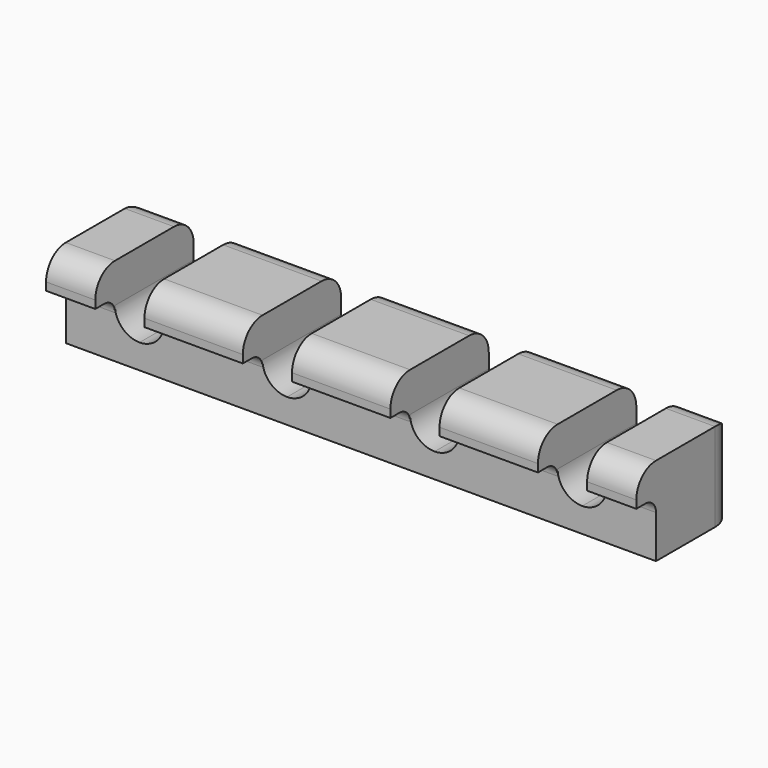
from build123d import *

# Parameters (mm, degrees)
F0_W      = 76.2
F0_H      = 12.7
F1_DEPTH  = 3.175
F2_W      = 6.35
F2_H      = 12.7
F2_W_2    = 12.7
F3_DEPTH  = 8.255
F4_W      = 6.35
F4_H      = 4.191
F4_W_2    = 12.7
F5_DEPTH  = 3.175
F7_DEPTH  = 6.35
F9_DEPTH  = 12.7
F11_DEPTH = 12.7
F13_DEPTH = 12.7
F15_DEPTH = 6.35
F17_DEPTH = 12.7
F18_R     = 3.175


with BuildPart() as f1:
    # F0 (on Top) → F1 (new body)
    with BuildSketch(Plane.XY):
        with Locations((-12.1522513986, 0.3075693393)):
            Rectangle(F0_W, F0_H)
    extrude(amount=F1_DEPTH)

    # F2 (on face) → F3 (join)
    with BuildSketch(Plane.XY.offset(3.175)):
        with Locations((-47.0772513986, 0.3075693393)):
            Rectangle(F2_W, F2_H)
        with Locations((-31.2022513986, 0.3075693393)):
            Rectangle(F2_W_2, F2_H)
        with Locations((-12.1522513986, 0.3075693393)):
            Rectangle(F2_W_2, F2_H)
        with Locations((6.8977486014, 0.3075693393)):
            Rectangle(F2_W_2, F2_H)
        with Locations((22.7727486014, 0.3075693393)):
            Rectangle(F2_W, F2_H)
    extrude(amount=F3_DEPTH)

    # F4 (on face) → F5 (join)
    with BuildSketch(Plane.XZ.offset(6.0424306607)):
        with Locations((-47.0772513986, 9.3345)):
            Rectangle(F4_W, F4_H)
        with Locations((-31.2022513986, 9.3345)):
            Rectangle(F4_W_2, F4_H)
        with Locations((-12.1522513986, 9.3345)):
            Rectangle(F4_W_2, F4_H)
        with Locations((6.8977486014, 9.3345)):
            Rectangle(F4_W_2, F4_H)
        with Locations((22.7727486014, 9.3345)):
            Rectangle(F4_W, F4_H)
    extrude(amount=F5_DEPTH)

    # F6 (on face) → F7 (join)
    with BuildSketch(Plane.YZ.offset(25.9477486014)):
        with BuildLine():
            Line((-6.0424306607, 7.239), (-7.7569306607, 7.239))
            ThreePointArc((-7.7569306607, 7.239), (-6.5445960844, 6.7368345763), (-6.0424306607, 5.5245))
            Line((-6.0424306607, 5.5245), (-6.0424306607, 7.239))
        make_face()
    extrude(amount=-F7_DEPTH)

    # F8 (on face) → F9 (join)
    with BuildSketch(Plane.YZ.offset(13.2477486014)):
        with BuildLine():
            Line((-6.0424306607, 7.239), (-7.7569306607, 7.239))
            ThreePointArc((-7.7569306607, 7.239), (-6.5445960844, 6.7368345763), (-6.0424306607, 5.5245))
            Line((-6.0424306607, 5.5245), (-6.0424306607, 7.239))
        make_face()
    extrude(amount=-F9_DEPTH)

    # F10 (on face) → F11 (join)
    with BuildSketch(Plane.YZ.offset(-5.8022513986)):
        with BuildLine():
            Line((-6.0424306607, 7.239), (-7.7569306607, 7.239))
            ThreePointArc((-7.7569306607, 7.239), (-6.5445960844, 6.7368345763), (-6.0424306607, 5.5245))
            Line((-6.0424306607, 5.5245), (-6.0424306607, 7.239))
        make_face()
    extrude(amount=-F11_DEPTH)

    # F12 (on face) → F13 (join)
    with BuildSketch(Plane.YZ.offset(-24.8522513986)):
        with BuildLine():
            Line((-6.0424306607, 7.239), (-7.7569306607, 7.239))
            ThreePointArc((-7.7569306607, 7.239), (-6.5445960844, 6.7368345763), (-6.0424306607, 5.5245))
            Line((-6.0424306607, 5.5245), (-6.0424306607, 7.239))
        make_face()
    extrude(amount=-F13_DEPTH)

    # F14 (on face) → F15 (join)
    with BuildSketch(Plane.YZ.offset(-43.9022513986)):
        with BuildLine():
            Line((-6.0424306607, 7.239), (-7.7569306607, 7.239))
            ThreePointArc((-7.7569306607, 7.239), (-6.5445960844, 6.7368345763), (-6.0424306607, 5.5245))
            Line((-6.0424306607, 5.5245), (-6.0424306607, 7.239))
        make_face()
    extrude(amount=-F15_DEPTH)

    # F16 (on face) → F17 (join)
    with BuildSketch(Plane.XZ.offset(6.0424306607)):
        with BuildLine():
            ThreePointArc((-40.7272513986, 3.175), (-42.9723154288, 4.1049359697), (-43.9022513986, 6.35))
            Line((-43.9022513986, 6.35), (-43.9022513986, 5.5245))
            Line((-43.9022513986, 5.5245), (-43.9022513986, 3.175))
            Line((-43.9022513986, 3.175), (-40.7272513986, 3.175))
        make_face()
        with BuildLine():
            ThreePointArc((-37.5522513986, 6.35), (-38.4821873683, 4.1049359697), (-40.7272513986, 3.175))
            Line((-40.7272513986, 3.175), (-37.5522513986, 3.175))
            Line((-37.5522513986, 3.175), (-37.5522513986, 5.5245))
            Line((-37.5522513986, 5.5245), (-37.5522513986, 6.35))
        make_face()
        with BuildLine():
            Line((-24.8522513986, 6.35), (-24.8522513986, 5.5245))
            Line((-24.8522513986, 5.5245), (-24.8522513986, 3.175))
            Line((-24.8522513986, 3.175), (-21.6772513986, 3.175))
            ThreePointArc((-21.6772513986, 3.175), (-23.9223154288, 4.1049359697), (-24.8522513986, 6.35))
        make_face()
        with BuildLine():
            ThreePointArc((-18.5022513986, 6.35), (-19.4321873683, 4.1049359697), (-21.6772513986, 3.175))
            Line((-21.6772513986, 3.175), (-18.5022513986, 3.175))
            Line((-18.5022513986, 3.175), (-18.5022513986, 5.5245))
            Line((-18.5022513986, 5.5245), (-18.5022513986, 6.35))
        make_face()
        with BuildLine():
            Line((-5.8022513986, 6.35), (-5.8022513986, 5.5245))
            Line((-5.8022513986, 5.5245), (-5.8022513986, 3.175))
            Line((-5.8022513986, 3.175), (-2.6272513986, 3.175))
            ThreePointArc((-2.6272513986, 3.175), (-4.8723154288, 4.1049359697), (-5.8022513986, 6.35))
        make_face()
        with BuildLine():
            Line((0.5477486014, 3.175), (0.5477486014, 5.5245))
            Line((0.5477486014, 5.5245), (0.5477486014, 6.35))
            ThreePointArc((0.5477486014, 6.35), (-0.3821873683, 4.1049359697), (-2.6272513986, 3.175))
            Line((-2.6272513986, 3.175), (0.5477486014, 3.175))
        make_face()
        with BuildLine():
            Line((13.2477486014, 3.175), (16.4227486014, 3.175))
            ThreePointArc((16.4227486014, 3.175), (14.1776845712, 4.1049359697), (13.2477486014, 6.35))
            Line((13.2477486014, 6.35), (13.2477486014, 5.5245))
            Line((13.2477486014, 5.5245), (13.2477486014, 3.175))
        make_face()
        with BuildLine():
            Line((19.5977486014, 3.175), (19.5977486014, 5.5245))
            Line((19.5977486014, 5.5245), (19.5977486014, 6.35))
            ThreePointArc((19.5977486014, 6.35), (18.6678126317, 4.1049359697), (16.4227486014, 3.175))
            Line((16.4227486014, 3.175), (19.5977486014, 3.175))
        make_face()
    extrude(amount=-F17_DEPTH)

    # F18
    f18_edges = [f1.edges().sort_by_distance(p)[0] for p in [
        (22.772749, 6.657569, 11.43),
        (6.897749, 6.657569, 11.43),
        (-12.152251, 6.657569, 11.43),
        (-31.202251, 6.657569, 11.43),
        (-47.077251, 6.657569, 11.43),
        (-47.077251, -9.217431, 11.43),
        (-31.202251, -9.217431, 11.43),
        (-12.152251, -9.217431, 11.43),
        (6.897749, -9.217431, 11.43),
        (22.772749, -9.217431, 11.43),
        (-50.252251, 6.657569, 5.715),
        (25.947749, 6.657569, 5.715),
    ]]
    fillet(f18_edges, radius=F18_R)


solid = f1.part
